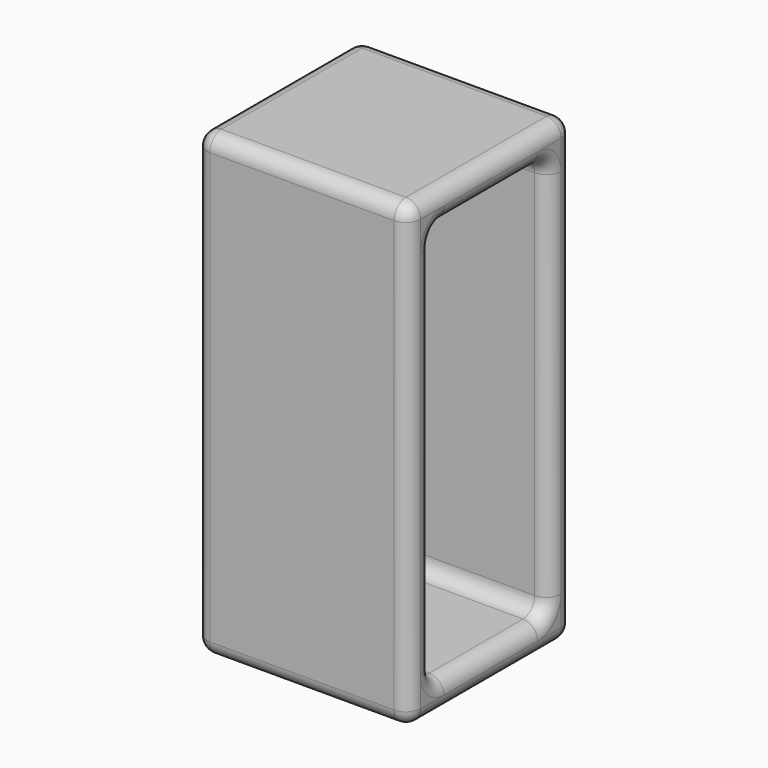
from build123d import *

# Parameters (mm, degrees)
F0_W     = 18.5276605189
F0_H     = 39.9128235877
F1_DEPTH = 17.78
F2_T     = -2.54
F3_R     = 1.26999


# Not quite as in the source:
# - a fillet or chamfer is up to 0.001 mm smaller than in the source, because OpenCascade refuses the exact size


with BuildPart() as f1:
    # F0 (on Front) → F1 (new body)
    with BuildSketch(Plane.XZ):
        with Locations((9.2638302594, 19.9564117938)):
            Rectangle(F0_W, F0_H)
    extrude(amount=F1_DEPTH)

    # F2
    f2_openings = [f1.faces().sort_by_distance(p)[0] for p in [
        (18.527661, -8.89, 19.956412),
    ]]
    offset(amount=F2_T, openings=f2_openings)

    # F3 (radius 1.27 in the source; OpenCascade refuses exactly that, so slightly less here)
    f3_edges = [f1.edges().sort_by_distance(p)[0] for p in [
        (18.527661, 0, 19.956412),
        (18.527661, -2.54, 19.956412),
        (18.527661, -8.89, 37.372824),
        (18.527661, -8.89, 39.912824),
        (18.527661, -15.24, 19.956412),
        (18.527661, -17.78, 19.956412),
        (18.527661, -8.89, 2.54),
        (18.527661, -8.89, 0),
        (9.26383, 0, 39.912824),
        (0, -8.89, 39.912824),
        (9.26383, -17.78, 39.912824),
        (2.54, -15.24, 19.956412),
        (2.54, -8.89, 2.54),
        (0, 0, 19.956412),
        (9.26383, 0, 0),
        (0, -17.78, 19.956412),
        (0, -8.89, 0),
        (9.26383, -17.78, 0),
        (2.54, -2.54, 19.956412),
        (10.53383, -2.54, 37.372824),
        (2.54, -8.89, 37.372824),
        (10.53383, -2.54, 2.54),
        (10.53383, -15.24, 2.54),
        (10.53383, -15.24, 37.372824),
    ]]
    fillet(f3_edges, radius=F3_R)


solid = f1.part
